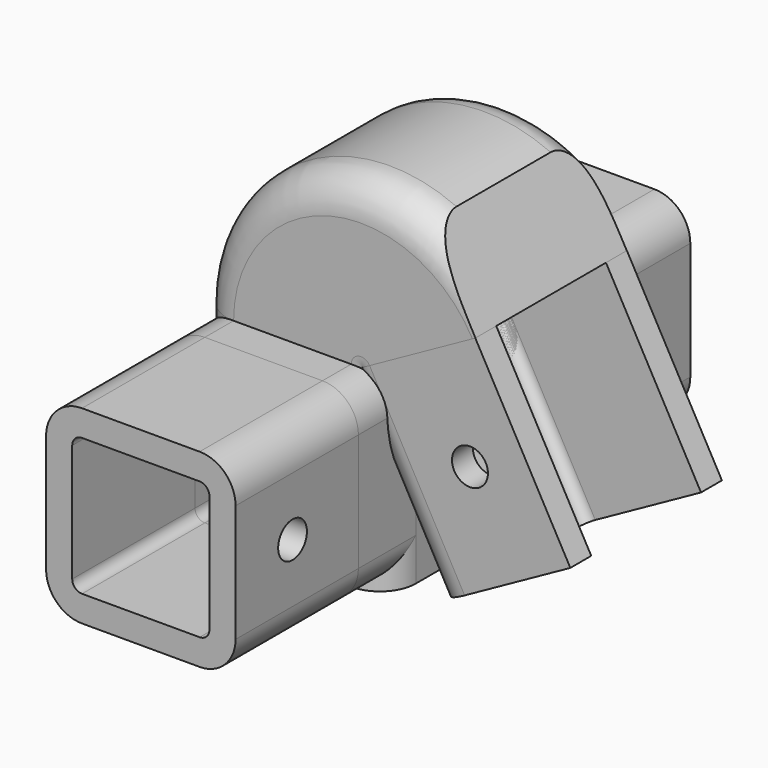
from build123d import *

# Parameters (mm, degrees)
F1_DEPTH  = 30
F3_DEPTH  = 21
F5_DEPTH  = 30
F7_DEPTH  = 30
F9_ANGLE  = 151
F11_DEPTH = 41
F13_DEPTH = 28
F15_DEPTH = 25
F17_DEPTH = 10
F18_W     = 18
F18_H     = 4
F19_DEPTH = 5.5
F21_DEPTH = 30
F23_DEPTH = 30
F25_DEPTH = 23.5
F30_R     = 2.75
F31_DEPTH = 5
F32_R     = 2.75
F33_DEPTH = 5


# Not quite as in the source:
# - a feature of the source that left no trace in its solid (it failed there, or was rolled back) is left out
# - a feature names something its author has since deleted; it is built from what else it names


with BuildPart() as f1:
    # F0 (on Top) → F1 (new body)
    with BuildSketch(Plane.XY):
        with BuildLine():
            Line((4, 1.5), (4, 19.5))
            ThreePointArc((4, 19.5), (2.3890872965, 23.3890872965), (-1.5, 25))
            Line((-1.5, 25), (-19.5, 25))
            ThreePointArc((-19.5, 25), (-23.3890872965, 23.3890872965), (-25, 19.5))
            Line((-25, 19.5), (-25, 1.5))
            ThreePointArc((-25, 1.5), (-23.3890872965, -2.3890872965), (-19.5, -4))
            Line((-19.5, -4), (-1.5, -4))
            ThreePointArc((-1.5, -4), (2.3890872965, -2.3890872965), (4, 1.5))
        make_face()
        with BuildLine():
            ThreePointArc((0, 1.5), (-0.4393398282, 0.4393398282), (-1.5, 0))
            Line((-1.5, 0), (-19.5, 0))
            ThreePointArc((-19.5, 0), (-20.5606601718, 0.4393398282), (-21, 1.5))
            Line((-21, 1.5), (-21, 19.5))
            ThreePointArc((-21, 19.5), (-20.5606601718, 20.5606601718), (-19.5, 21))
            Line((-19.5, 21), (-1.5, 21))
            ThreePointArc((-1.5, 21), (-0.4393398282, 20.5606601718), (0, 19.5))
            Line((0, 19.5), (0, 1.5))
        make_face(mode=Mode.SUBTRACT)
    extrude(amount=-F1_DEPTH)

    # F2 (on Front) → F3 (join)
    with BuildSketch(Plane.XZ):
        Polygon((17.4923941428, 9.6961924049), (0, 0), (14.5442886074, -26.2385912142), (32.0366827502, -16.5423988093), align=None)
    extrude(amount=-F3_DEPTH)

    # F4 (on face) → F5 (join)
    with BuildSketch(Plane(origin=(14.5442886074, 0, -26.2385912142), x_dir=(0.8746197071, 0, 0.4848096202), z_dir=(0.4848096202, 0, -0.8746197071))):
        with BuildLine():
            Line((1.5, 0), (20, 0))
            Line((20, 0), (20, 4))
            Line((20, 4), (1.5, 4))
            ThreePointArc((1.5, 4), (-2.3890872965, 2.3890872965), (-4, -1.5))
            Line((-4, -1.5), (-4, -19.5))
            ThreePointArc((-4, -19.5), (-2.3890872965, -23.3890872965), (1.5, -25))
            Line((1.5, -25), (20, -25))
            Line((20, -25), (20, -21))
            Line((20, -21), (1.5, -21))
            Line((1.5, -21), (0, -21))
            Line((0, -21), (0, -19.5))
            Line((0, -19.5), (0, -1.5))
            Line((0, -1.5), (0, 0))
            Line((0, 0), (1.5, 0))
        make_face()
    extrude(amount=-F5_DEPTH)

    # F6 (on face) → F7 (cut)
    with BuildSketch(Plane(origin=(14.5442886074, 0, -26.2385912142), x_dir=(0.8746197071, 0, 0.4848096202), z_dir=(0.4848096202, 0, -0.8746197071))):
        with BuildLine():
            Line((20, -21), (20, 0))
            Line((20, 0), (1.5, 0))
            ThreePointArc((1.5, 0), (0.4393398282, -0.4393398282), (0, -1.5))
            Line((0, -1.5), (0, -19.5))
            ThreePointArc((0, -19.5), (0.4393398282, -20.5606601718), (1.5, -21))
            Line((1.5, -21), (20, -21))
        make_face()
    extrude(amount=-F7_DEPTH, mode=Mode.SUBTRACT)

    # F12 (on face) → F13 (cut)
    with BuildSketch(Plane(origin=(0, 0, -30), x_dir=(1, 0, 0), z_dir=(0, 0, -1))):
        with BuildLine():
            Line((-9, -21), (-1.5, -21))
            ThreePointArc((-1.5, -21), (-0.4393398282, -20.5606601718), (0, -19.5))
            Line((0, -19.5), (0, -1.5))
            ThreePointArc((0, -1.5), (-0.4393398282, -0.4393398282), (-1.5, 0))
            Line((-1.5, 0), (-9, 0))
            ThreePointArc((-9, 0), (-10.0606601718, -0.4393398282), (-10.5, -1.5))
            Line((-10.5, -1.5), (-10.5, -19.5))
            ThreePointArc((-10.5, -19.5), (-10.0606601718, -20.5606601718), (-9, -21))
        make_face()
    extrude(amount=-F13_DEPTH, mode=Mode.SUBTRACT)

    # F14 (on face) → F15 (cut)
    with BuildSketch(Plane.XZ.offset(4)):
        with BuildLine():
            ThreePointArc((19.4243061554, -7.9075921894), (18.0700366536, -5.5381119982), (15.3410796998, -5.5023879948))
            Line((15.3410796998, -5.5023879948), (18.0075326111, -10.3127963841))
            ThreePointArc((18.0075326111, -10.3127963841), (19.0437863467, -9.3033226876), (19.4243061554, -7.9075921894))
        make_face()
        with BuildLine():
            Line((18.0075326111, -10.3127963841), (15.3410796998, -5.5023879948))
            ThreePointArc((15.3410796998, -5.5023879948), (14.2691019608, -9.2408186451), (18.0075326111, -10.3127963841))
        make_face()
    extrude(amount=-F15_DEPTH, mode=Mode.SUBTRACT)

    # F16 (on face) → F17 (cut)
    with BuildSketch(Plane.XZ.offset(4)):
        with BuildLine():
            ThreePointArc((-7.75, -15), (-8.5554563517, -13.0554563517), (-10.5, -12.25))
            Line((-10.5, -12.25), (-10.5, -17.75))
            ThreePointArc((-10.5, -17.75), (-8.5554563517, -16.9445436483), (-7.75, -15))
        make_face()
        with BuildLine():
            Line((-10.5, -17.75), (-10.5, -12.25))
            ThreePointArc((-10.5, -12.25), (-13.25, -15), (-10.5, -17.75))
        make_face()
    extrude(amount=-F17_DEPTH, mode=Mode.SUBTRACT)


with BuildPart() as f9:
    # F8 (on face) → F9 (revolve)
    with BuildSketch(Plane.XY):
        with BuildLine():
            ThreePointArc((-21, 19.5), (-20.5606601718, 20.5606601718), (-19.5, 21))
            Line((-19.5, 21), (-1.5, 21))
            ThreePointArc((-1.5, 21), (-0.4393398282, 20.5606601718), (0, 19.5))
            Line((0, 19.5), (0, 24.7915026221))
            ThreePointArc((0, 24.7915026221), (-0.7427894684, 24.9476262914), (-1.5, 25))
            Line((-1.5, 25), (-19.5, 25))
            ThreePointArc((-19.5, 25), (-23.3890872965, 23.3890872965), (-25, 19.5))
            Line((-25, 19.5), (-25, 1.5))
            ThreePointArc((-25, 1.5), (-23.3890872965, -2.3890872965), (-19.5, -4))
            Line((-19.5, -4), (-1.5, -4))
            ThreePointArc((-1.5, -4), (-0.7427894684, -3.9476262914), (0, -3.7915026221))
            Line((0, -3.7915026221), (0, 1.5))
            ThreePointArc((0, 1.5), (-0.4393398282, 0.4393398282), (-1.5, 0))
            Line((-1.5, 0), (-19.5, 0))
            ThreePointArc((-19.5, 0), (-20.5606601718, 0.4393398282), (-21, 1.5))
            Line((-21, 1.5), (-21, 19.5))
        make_face()
        with BuildLine():
            Line((-1.5, 21), (-19.5, 21))
            ThreePointArc((-19.5, 21), (-20.5606601718, 20.5606601718), (-21, 19.5))
            Line((-21, 19.5), (-21, 1.5))
            ThreePointArc((-21, 1.5), (-20.5606601718, 0.4393398282), (-19.5, 0))
            Line((-19.5, 0), (-1.5, 0))
            ThreePointArc((-1.5, 0), (-0.4393398282, 0.4393398282), (0, 1.5))
            Line((0, 1.5), (0, 19.5))
            ThreePointArc((0, 19.5), (-0.4393398282, 20.5606601718), (-1.5, 21))
        make_face()
    revolve(axis=Axis((0, 10.5, 0), (0, 1, 0)), revolution_arc=F9_ANGLE)

    # F10 (on face) → F11 (cut)
    with BuildSketch(Plane(origin=(0, 25, 0), x_dir=(-1, 0, 0), z_dir=(0, 1, 0))):
        Polygon((-34.1248847544, 7.7525814995), (-17.4923941428, 9.6961924049), (-8.9943257545, 25.027113605), align=None)
    extrude(amount=-F11_DEPTH, mode=Mode.SUBTRACT)


with BuildPart() as f19:
    # F18 (on face) → F19 (new body, symmetric)
    with BuildSketch(Plane(origin=(0, 25, 0), x_dir=(-1, 0, 0), z_dir=(0, 1, 0))):
        with BuildLine():
            ThreePointArc((-4, -23.5), (-2.3890872965, -27.3890872965), (1.5, -29))
            Line((1.5, -29), (1.5, -25))
            ThreePointArc((1.5, -25), (0.4393398282, -24.5606601718), (0, -23.5))
            Line((0, -23.5), (0, -5.5))
            ThreePointArc((0, -5.5), (0.4393398282, -4.4393398282), (1.5, -4))
            Line((1.5, -4), (1.5, 0))
            ThreePointArc((1.5, 0), (-2.3890872965, -1.6109127035), (-4, -5.5))
            Line((-4, -5.5), (-4, -23.5))
        make_face()
        with Locations((10.5, -2)):
            Rectangle(F18_W, F18_H)
        with BuildLine():
            Line((19.5, -25), (19.5, -29))
            ThreePointArc((19.5, -29), (23.3890872965, -27.3890872965), (25, -23.5))
            Line((25, -23.5), (25, -5.5))
            ThreePointArc((25, -5.5), (23.3890872965, -1.6109127035), (19.5, 0))
            Line((19.5, 0), (19.5, -4))
            ThreePointArc((19.5, -4), (20.5606601718, -4.4393398282), (21, -5.5))
            Line((21, -5.5), (21, -23.5))
            ThreePointArc((21, -23.5), (20.5606601718, -24.5606601718), (19.5, -25))
        make_face()
        with Locations((10.5, -27)):
            Rectangle(F18_W, F18_H)
    extrude(amount=F19_DEPTH, both=True)


with BuildPart() as f21_tool:
    # F20 (on face) → F21 (new body)
    with BuildSketch(Plane(origin=(0, 0, -30), x_dir=(1, 0, 0), z_dir=(0, 0, -1))):
        with BuildLine():
            Line((-19.5, -21), (-1.5, -21))
            ThreePointArc((-1.5, -21), (-0.4393398282, -20.5606601718), (0, -19.5))
            Line((0, -19.5), (0, -1.5))
            ThreePointArc((0, -1.5), (-0.4393398282, -0.4393398282), (-1.5, 0))
            Line((-1.5, 0), (-19.5, 0))
            ThreePointArc((-19.5, 0), (-20.5606601718, -0.4393398282), (-21, -1.5))
            Line((-21, -1.5), (-21, -19.5))
            ThreePointArc((-21, -19.5), (-20.5606601718, -20.5606601718), (-19.5, -21))
        make_face()
    extrude(amount=-F21_DEPTH)


with BuildPart() as f1_1:
    add(f1.part)

    # F21: cut by f21_tool
    add(f21_tool.part, mode=Mode.SUBTRACT)


with BuildPart() as f19_1:
    add(f19.part)

    # F21: cut by f21_tool
    add(f21_tool.part, mode=Mode.SUBTRACT)

    # F22 (on face) → F23 (cut)
    with BuildSketch(Plane(origin=(14.5442886074, 0, -26.2385912142), x_dir=(0.8746197071, 0, 0.4848096202), z_dir=(0.4848096202, 0, -0.8746197071))):
        with BuildLine():
            Line((3.0479622073, -19.5), (0, -19.5))
            ThreePointArc((0, -19.5), (0.4393398282, -20.5606601718), (1.5, -21))
            Line((1.5, -21), (3.0479622073, -21))
            Line((3.0479622073, -21), (3.0479622073, -19.5))
        make_face()
    extrude(amount=-F23_DEPTH, mode=Mode.SUBTRACT)


with BuildPart() as f25:
    # F24 (on face) → F25 (new body)
    with BuildSketch(Plane(origin=(0, 30.5, 0), x_dir=(-1, 0, 0), z_dir=(0, 1, 0))):
        with BuildLine():
            Line((1.5, -29), (19.5, -29))
            ThreePointArc((19.5, -29), (23.3890872965, -27.3890872965), (25, -23.5))
            Line((25, -23.5), (25, -5.5))
            ThreePointArc((25, -5.5), (23.3890872965, -1.6109127035), (19.5, 0))
            Line((19.5, 0), (1.5, 0))
            ThreePointArc((1.5, 0), (-2.3890872965, -1.6109127035), (-4, -5.5))
            Line((-4, -5.5), (-4, -23.5))
            ThreePointArc((-4, -23.5), (-2.3890872965, -27.3890872965), (1.5, -29))
        make_face()
        with BuildLine():
            Line((1.5, -4), (19.5, -4))
            ThreePointArc((19.5, -4), (20.5606601718, -4.4393398282), (21, -5.5))
            Line((21, -5.5), (21, -23.5))
            ThreePointArc((21, -23.5), (20.5606601718, -24.5606601718), (19.5, -25))
            Line((19.5, -25), (1.5, -25))
            ThreePointArc((1.5, -25), (0.4393398282, -24.5606601718), (0, -23.5))
            Line((0, -23.5), (0, -5.5))
            ThreePointArc((0, -5.5), (0.4393398282, -4.4393398282), (1.5, -4))
        make_face(mode=Mode.SUBTRACT)
    extrude(amount=F25_DEPTH)


with BuildPart() as f29_1:
    # F29: instance of F19
    add(f19_1.part.mirror(Plane.XZ.offset(-10.5)))


with BuildPart() as f29_2:
    # F29: instance of F25
    add(f25.part.mirror(Plane.XZ.offset(-10.5)))

    # F32 (on face) → F33 (cut)
    with BuildSketch(Plane.YZ.offset(4)):
        with Locations((-22.0986865461, -14.5)):
            Circle(F32_R)
    extrude(amount=-F33_DEPTH, mode=Mode.SUBTRACT)


with BuildPart() as f25_1:
    add(f25.part)

    # F30 (on face) → F31 (cut)
    with BuildSketch(Plane.YZ.offset(4)):
        with Locations((42.0185364783, -14.5)):
            Circle(F30_R)
    extrude(amount=-F31_DEPTH, mode=Mode.SUBTRACT)


solid = Compound([f9.part, f1_1.part, f19_1.part, f29_1.part, f29_2.part, f25_1.part])
